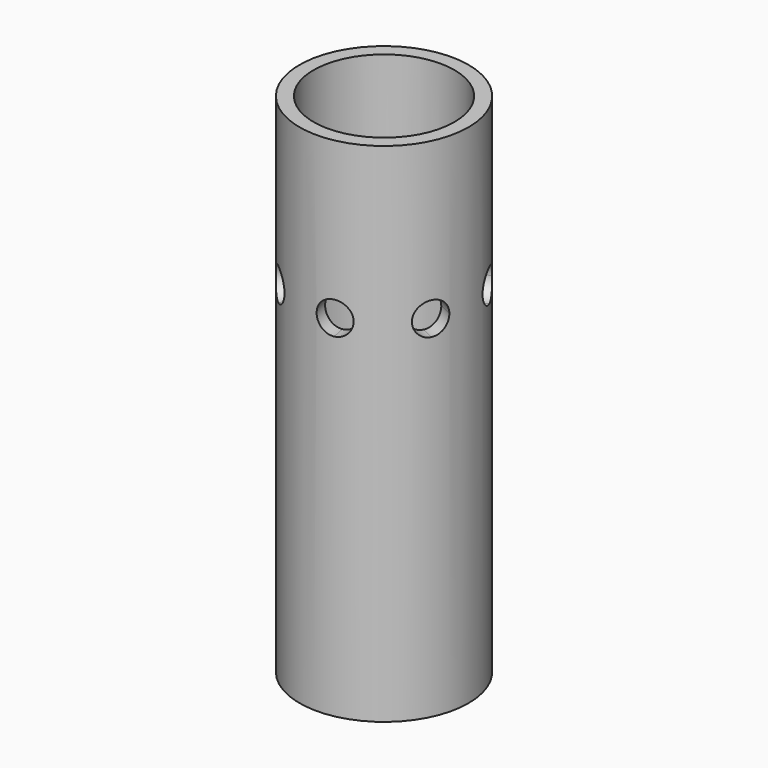
from build123d import *

# Parameters (mm, degrees)
F0_R      = 19.05
F1_DEPTH  = 109.474
F2_R      = 15.873592274
F3_DEPTH  = 109.728
F4_R      = 19.05
F5_DEPTH  = 1.27
F25_DEPTH = 25.4
F26_DEPTH = 32.004
F28_DEPTH = 45.466
F30_DEPTH = 34.036
F32_DEPTH = 25.4
F34_DEPTH = 25.4
F36_DEPTH = 53.086
F38_DEPTH = 65.786
F39_R     = 19.05
F40_DEPTH = 4.826
F41_R     = 16.1364398947
F41_R_2   = 15.139722271
F42_DEPTH = 1.27
F43_SIZE  = 0.254
F44_R     = 8.561127958
F44_R_2   = 8.1224197416
F45_DEPTH = 0.508


with BuildPart() as f1:
    # F0 (on Top) → F1 (new body)
    with BuildSketch(Plane.XY):
        Circle(F0_R)
    extrude(amount=F1_DEPTH)

    # F2 (on face) → F3 (cut)
    with BuildSketch(Plane.XY.offset(109.474)):
        Circle(F2_R)
    extrude(amount=-F3_DEPTH, mode=Mode.SUBTRACT)

    # F4 (on Top) → F5 (join)
    with BuildSketch(Plane.XY):
        Circle(F4_R)
    extrude(amount=-F5_DEPTH)

    # F24 (on face) → F25 (join)
    with BuildSketch(Plane(origin=(0, 0, 0), x_dir=(0.4275550934, 0.9039892931, 0), z_dir=(0.9039892931, -0.4275550934, 0))):
        with BuildLine():
            ThreePointArc((0, 70.5485), (2.595294019, 71.623505981), (3.6703, 74.2188))
            ThreePointArc((3.6703, 74.2188), (-2.595294019, 76.814094019), (0, 70.5485))
        make_face()
    extrude(amount=F25_DEPTH)

    # F26 (cut): a face of the model
    f26_faces = [f1.faces().sort_by_distance(p)[0] for p in [
        (22.9613280453, -10.8598993731, 74.2188),
    ]]
    extrude(f26_faces, amount=-F26_DEPTH, mode=Mode.SUBTRACT)

    # F27 (on face) → F28 (cut)
    with BuildSketch(Plane(origin=(0, 0, 0), x_dir=(-0.4275550934, 0.9039892931, 0), z_dir=(0.9039892931, 0.4275550934, 0))):
        with BuildLine():
            ThreePointArc((0, 70.5485), (2.595294019, 71.623505981), (3.6703, 74.2188))
            ThreePointArc((3.6703, 74.2188), (-2.595294019, 76.814094019), (0, 70.5485))
        make_face()
    extrude(amount=F28_DEPTH, mode=Mode.SUBTRACT)

    # F29 (on face) → F30 (cut)
    with BuildSketch(Plane(origin=(0, 0, 0), x_dir=(0.9700312532, -0.2429801799, 0), z_dir=(-0.2429801799, -0.9700312532, 0))):
        with BuildLine():
            ThreePointArc((0, 70.5485), (2.595294019, 71.623505981), (3.6703, 74.2188))
            ThreePointArc((3.6703, 74.2188), (-2.595294019, 76.814094019), (0, 70.5485))
        make_face()
    extrude(amount=-F30_DEPTH, mode=Mode.SUBTRACT)

    # F31 (on face) → F32 (cut)
    with BuildSketch(Plane(origin=(0, 0, 0), x_dir=(0.7730104534, 0.6343932842, 0), z_dir=(0.6343932842, -0.7730104534, 0))):
        with BuildLine():
            ThreePointArc((0, 70.5485), (2.595294019, 71.623505981), (3.6703, 74.2188))
            ThreePointArc((3.6703, 74.2188), (-2.595294019, 76.814094019), (0, 70.5485))
        make_face()
    extrude(amount=-F32_DEPTH, mode=Mode.SUBTRACT)

    # F33 (on Right) → F34 (cut)
    with BuildSketch(Plane.YZ):
        with BuildLine():
            ThreePointArc((0, 70.5485), (2.595294019, 71.623505981), (3.6703, 74.2188))
            ThreePointArc((3.6703, 74.2188), (-2.595294019, 76.814094019), (0, 70.5485))
        make_face()
    extrude(amount=-F34_DEPTH, mode=Mode.SUBTRACT)

    # F35 (on face) → F36 (cut)
    with BuildSketch(Plane(origin=(0, 0, 0), x_dir=(0.7730104534, -0.6343932842, 0), z_dir=(-0.6343932842, -0.7730104534, 0))):
        with BuildLine():
            ThreePointArc((0, 70.5485), (2.595294019, 71.623505981), (3.6703, 74.2188))
            ThreePointArc((3.6703, 74.2188), (-2.595294019, 76.814094019), (0, 70.5485))
        make_face()
    extrude(amount=F36_DEPTH, mode=Mode.SUBTRACT)

    # F37 (on face) → F38 (cut)
    with BuildSketch(Plane(origin=(0, 0, 0), x_dir=(0.9807852804, 0.195090322, 0), z_dir=(0.195090322, -0.9807852804, 0))):
        with BuildLine():
            ThreePointArc((0, 70.5485), (2.595294019, 71.623505981), (3.6703, 74.2188))
            ThreePointArc((3.6703, 74.2188), (-2.595294019, 76.814094019), (0, 70.5485))
        make_face()
    extrude(amount=F38_DEPTH, mode=Mode.SUBTRACT)

    # F39 (on Top) → F40 (join)
    with BuildSketch(Plane.XY):
        Circle(F39_R)
    extrude(amount=-F40_DEPTH)

    # F41 (on face) → F42 (cut)
    with BuildSketch(Plane(origin=(0, 0, -4.826), x_dir=(1, 0, 0), z_dir=(0, 0, -1))):
        Circle(F41_R)
        Circle(F41_R_2, mode=Mode.SUBTRACT)
    extrude(amount=-F42_DEPTH, mode=Mode.SUBTRACT)

    # F43
    f43_edges = [f1.edges().sort_by_distance(p)[0] for p in [
        (-15.139722, 0, -3.556),
    ]]
    chamfer(f43_edges, length=F43_SIZE)

    # F44 (on face) → F45 (cut)
    with BuildSketch(Plane(origin=(0, 0, -4.826), x_dir=(1, 0, 0), z_dir=(0, 0, -1))):
        Circle(F44_R)
        Circle(F44_R_2, mode=Mode.SUBTRACT)
    extrude(amount=-F45_DEPTH, mode=Mode.SUBTRACT)


solid = f1.part
